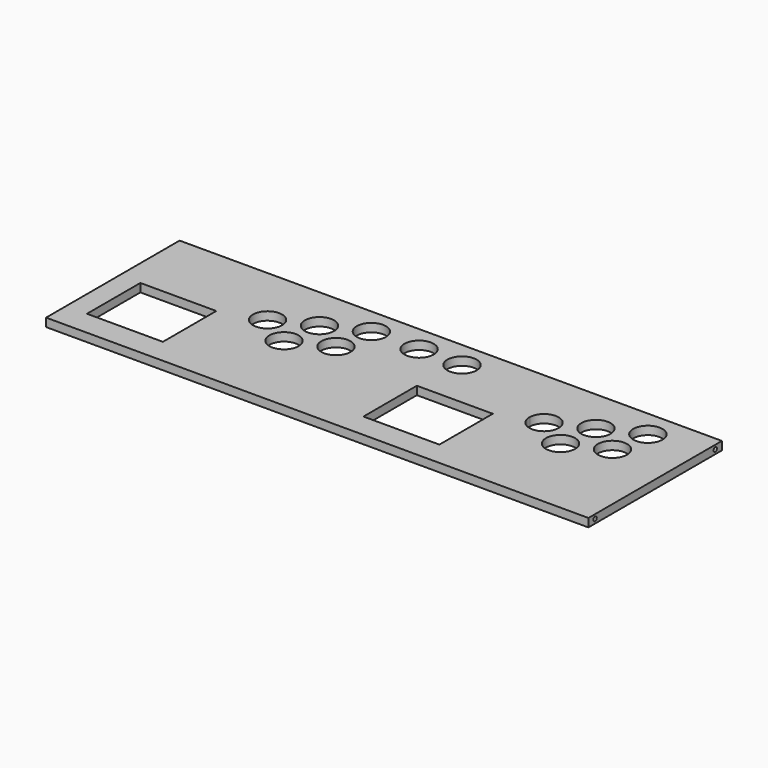
from build123d import *

# Parameters (mm, degrees)
F0_W           = 650
F0_H           = 200
F1_DEPTH       = 10
F4_D           = 5
F4_DEPTH       = 20
F4_TIP         = 1.5021515476
F4_ON_F3_D     = 5
F4_ON_F3_DEPTH = 20
F4_ON_F3_TIP   = 1.5021515476
F5_W           = 91
F5_H           = 80
F6_DEPTH       = 25


with BuildPart() as f1:
    # F0 (on Top) → F1 (new body)
    with BuildSketch(Plane.XY):
        Rectangle(F0_W, F0_H)
    extrude(amount=F1_DEPTH)

    # F4
    with Locations(Plane.YZ.offset(325)):
        with Locations((90, 5), (-90, 5)):
            Hole(F4_D / 2, depth=F4_DEPTH)
            with Locations((0, 0, -(F4_DEPTH + F4_TIP / 2))):  # 118° drill point
                Cone(0, F4_D / 2, F4_TIP, mode=Mode.SUBTRACT)

    # F4 on F3
    with Locations(Plane(origin=(-325, 0, 0), x_dir=(0, -1, 0), z_dir=(-1, 0, 0))):
        with Locations((90, 5), (-90, 5)):
            Hole(F4_ON_F3_D / 2, depth=F4_ON_F3_DEPTH)
            with Locations((0, 0, -(F4_ON_F3_DEPTH + F4_ON_F3_TIP / 2))):  # 118° drill point
                Cone(0, F4_ON_F3_D / 2, F4_ON_F3_TIP, mode=Mode.SUBTRACT)

    # F5 (on face) → F6 (cut)
    with BuildSketch(Plane.XY.offset(10)):
        with BuildLine():
            ThreePointArc((-144.4550033747, 33.3169048253), (-167.7112094275, 41.7814723445), (-176.1757760637, 18.5252659703))
            ThreePointArc((-176.1757760637, 18.5252659703), (-152.9195705725, 10.0606996555), (-144.4550033747, 33.3169048253))
        make_face()
        with BuildLine():
            ThreePointArc((-99.1396139363, 54.4478180297), (-122.3958194275, 62.9123843445), (-130.8603866253, 39.6561791747))
            ThreePointArc((-130.8603866253, 39.6561791747), (-107.6041805725, 31.1916116555), (-99.1396139363, 54.4478180297))
        make_face()
        with BuildLine():
            ThreePointArc((-60.6337345533, 31.0267332083), (-83.889940619, 39.4913002552), (-92.3545070637, 16.2350939703))
            ThreePointArc((-92.3545070637, 16.2350939703), (-69.098301381, 7.7705277448), (-60.6337345533, 31.0267332083))
        make_face()
        with BuildLine():
            ThreePointArc((-105.9491247577, 9.8958196467), (-129.2053308382, 18.360386153), (-137.6698970637, -4.8958200297))
            ThreePointArc((-137.6698970637, -4.8958200297), (-114.4136911618, -13.360386153), (-105.9491247577, 9.8958196467))
        make_face()
        with BuildLine():
            ThreePointArc((-53.8242245533, 75.5787312083), (-77.080430619, 84.0432982552), (-85.5449970637, 60.7870919703))
            ThreePointArc((-85.5449970637, 60.7870919703), (-62.288791381, 52.3225257448), (-53.8242245533, 75.5787312083))
        make_face()
        with Locations((-254.5, -30)):
            Rectangle(F5_W, F5_H)
        with BuildLine():
            ThreePointArc((189.369221, 24.921086), (188.954401169, 28.7087790435), (187.7296074467, 32.3169052083))
            ThreePointArc((187.7296074467, 32.3169052083), (168.3260134713, 42.0586377624), (154.3763653155, 25.421086))
            ThreePointArc((154.3763653155, 25.421086), (154.7316693294, 21.3778780275), (156.0088349363, 17.5252659703))
            ThreePointArc((156.0088349363, 17.5252659703), (175.6569144859, 7.835905929), (189.369221, 24.921086))
        make_face()
        with BuildLine():
            ThreePointArc((233.0449962423, 53.4478176467), (209.7887905725, 61.9123843445), (201.3242235533, 38.6561787917))
            ThreePointArc((201.3242235533, 38.6561787917), (224.5804294275, 30.1916116555), (233.0449962423, 53.4478176467))
        make_face()
        with BuildLine():
            ThreePointArc((271.5508764467, 30.0267332083), (248.2946705725, 38.4913003445), (239.8301037577, 15.2350943533))
            ThreePointArc((239.8301037577, 15.2350943533), (263.0863094275, 6.7705276555), (271.5508764467, 30.0267332083))
        make_face()
        with BuildLine():
            ThreePointArc((226.2354870637, 8.8958200297), (202.9792811618, 17.360386153), (194.5147147577, -5.8958196467))
            ThreePointArc((194.5147147577, -5.8958196467), (217.7709208382, -14.360386153), (226.2354870637, 8.8958200297))
        make_face()
        with BuildLine():
            ThreePointArc((278.3603856253, 74.5787308253), (255.1041795725, 83.0432983445), (246.6396129363, 59.7870919703))
            ThreePointArc((246.6396129363, 59.7870919703), (269.8958184275, 51.3225256555), (278.3603856253, 74.5787308253))
        make_face()
        Polygon((32.18461, -70), (32.18461, -71), (123.18461, -71), (123.18461, -70), (123.18461, 9), (32.18461, 9), align=None)
        with BuildLine():
            ThreePointArc((5, 68.182912), (-12.5, 85.682912), (-30, 68.182912))
            ThreePointArc((-30, 68.182912), (-12.5, 50.682912), (5, 68.182912))
        make_face()
        with BuildLine():
            ThreePointArc((56.428404, 68.182912), (38.928404, 85.682912), (21.428404, 68.182912))
            ThreePointArc((21.428404, 68.182912), (38.928404, 50.682912), (56.428404, 68.182912))
        make_face()
    extrude(amount=-F6_DEPTH, mode=Mode.SUBTRACT)


solid = f1.part
